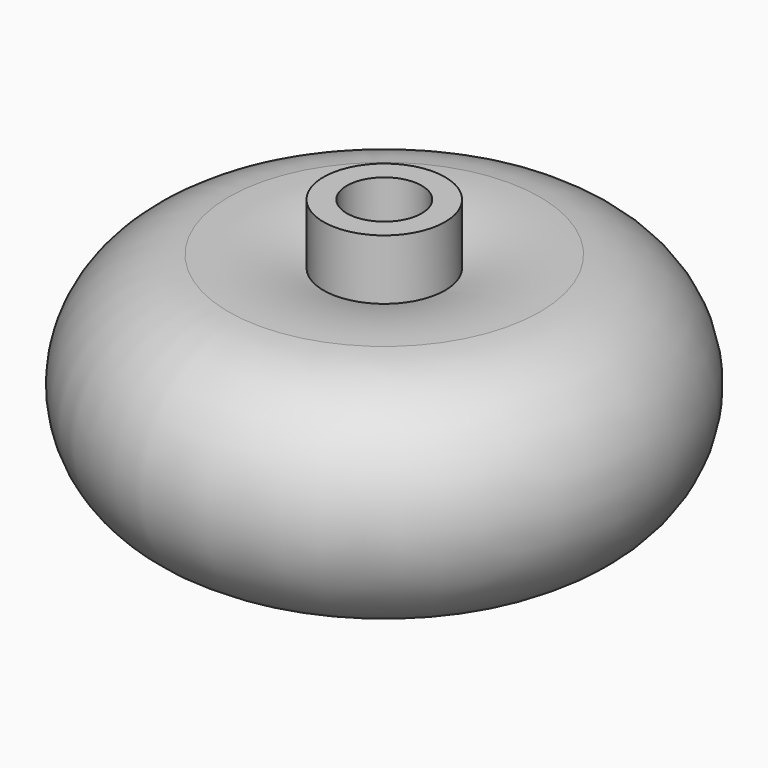
from build123d import *

# Parameters (mm, degrees)
F2_R        = 4.699
F3_DEPTH    = 9.525
F4_R        = 2.2225
F1_FACE_R   = 7.62
F1_FACE_R_2 = 4.699
F5_DEPTH    = 22.225


# Not quite as in the source:
# - a feature names something its author has since deleted; it is built from what else it names


with BuildPart() as f1:
    # F0 (on Front) → F1 (revolve)
    with BuildSketch(Plane.XZ):
        with BuildLine():
            ThreePointArc((11.0330758616, -81.8918719888), (13.2853990557, -80.4988733509), (15.6419463456, -79.2905315757))
            ThreePointArc((15.6419463456, -79.2905315757), (32.9902043329, -67.2816433685), (19.5133984089, -51.0473847389))
            ThreePointArc((19.5133984089, -51.0473847389), (13.498708034, -51.2466242985), (7.62, -52.533864975))
            Line((7.62, -52.533864975), (7.62, -44.9823363346))
            Line((7.62, -44.9823363346), (0, -44.9823363346))
            Line((0, -44.9823363346), (0, -88.1623363346))
            Line((0, -88.1623363346), (5.08, -88.1623363346))
            ThreePointArc((5.08, -88.1623363346), (5.7963291238, -86.1365407799), (7.512565547, -84.843672812))
            ThreePointArc((7.512565547, -84.843672812), (9.2048459257, -83.286701243), (11.0330758616, -81.8918719888))
        make_face()
    revolve(axis=Axis((0, 0, -66.5723363346), (0, 0, -1)))

    # F2 (on face) → F3 (cut)
    with BuildSketch(Plane.XY.offset(-44.9823363346)):
        Circle(F2_R)
    extrude(amount=-F3_DEPTH, mode=Mode.SUBTRACT)

    # F4 (on face) + F1_face (on face) → F5 (cut)
    with BuildSketch(Plane(origin=(0, 0, -88.1623363346), x_dir=(1, 0, 0), z_dir=(0, 0, -1))):
        Circle(F4_R)
    with BuildSketch(Plane.XY.offset(-44.9823363346)):
        Circle(F1_FACE_R)
        Circle(F1_FACE_R_2, mode=Mode.SUBTRACT)
    extrude(amount=-F5_DEPTH, dir=(0, 0, -1), mode=Mode.SUBTRACT)


solid = f1.part
